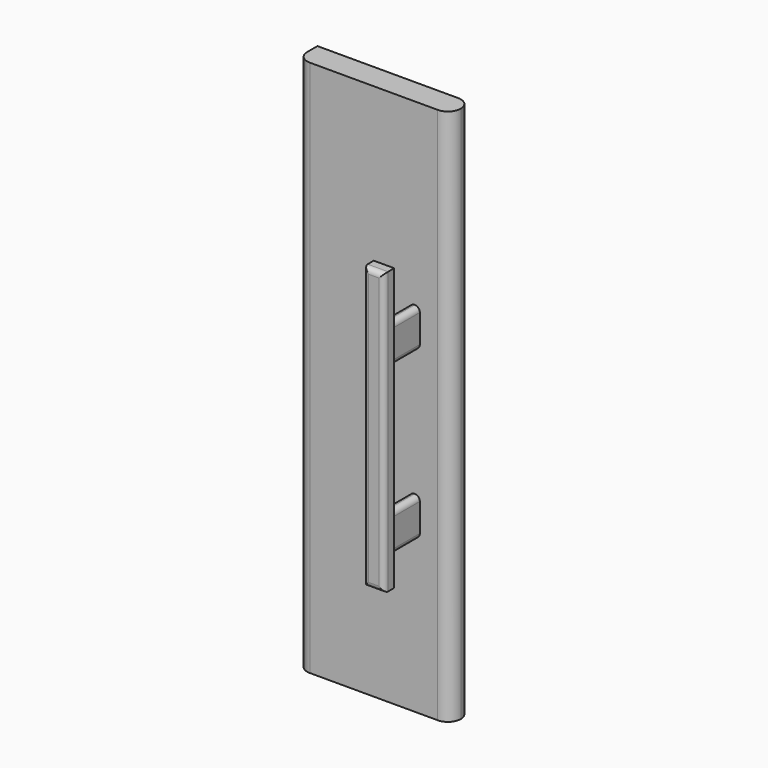
from build123d import *

# Parameters (mm, degrees)
F1_DEPTH = 533.4
F4_W     = 10.16
F4_H     = 38.1
F5_DEPTH = 38.1
F6_R     = 5.07999
F3_W     = 20.32
F3_H     = 279.4
F7_DEPTH = 12.7
F8_R     = 5.08


# Not quite as in the source:
# - a fillet or chamfer is up to 0.001 mm smaller than in the source, because OpenCascade refuses the exact size


with BuildPart() as f1:
    # F0 (on Top) → F1 (new body)
    with BuildSketch(Plane.XY):
        with BuildLine():
            Line((63.5, 25.4), (-76.2, 25.4))
            Line((-76.2, 25.4), (-76.2, 12.7))
            ThreePointArc((-76.2, 12.7), (-72.4802561211, 3.7197438789), (-63.5, 0))
            Line((-63.5, 0), (63.5, 0))
            ThreePointArc((63.5, 0), (72.4802561211, 3.7197438789), (76.2, 12.7))
            ThreePointArc((76.2, 12.7), (72.4802561211, 21.6802561211), (63.5, 25.4))
        make_face()
    extrude(amount=F1_DEPTH)

    # F4 (on face) → F5 (join, through all)
    with BuildSketch(Plane.XZ):
        with Locations((40.64, 336.55)):
            Rectangle(F4_W, F4_H)
        with Locations((40.64, 171.45)):
            Rectangle(F4_W, F4_H)
    extrude(amount=F5_DEPTH)

    # F6 (radius 5.08 in the source; OpenCascade refuses exactly that, so slightly less here)
    f6_edges = [f1.edges().sort_by_distance(p)[0] for p in [
        (35.56, -19.05, 355.6),
        (45.72, -19.05, 355.6),
        (45.72, -19.05, 317.5),
        (35.56, -19.05, 317.5),
        (35.56, -19.05, 190.5),
        (45.72, -19.05, 190.5),
        (35.56, -19.05, 152.4),
        (45.72, -19.05, 152.4),
    ]]
    fillet(f6_edges, radius=F6_R)

    # F3 (on offset) → F7 (join)
    with BuildSketch(Plane.XZ.offset(38.1)):
        with Locations((40.64, 266.7)):
            Rectangle(F3_W, F3_H)
    extrude(amount=F7_DEPTH)

    # F8
    f8_edges = [f1.edges().sort_by_distance(p)[0] for p in [
        (40.64, -50.8, 406.4),
        (30.48, -50.8, 266.7),
        (50.8, -50.8, 266.7),
        (40.64, -50.8, 127),
    ]]
    fillet(f8_edges, radius=F8_R)


solid = f1.part
